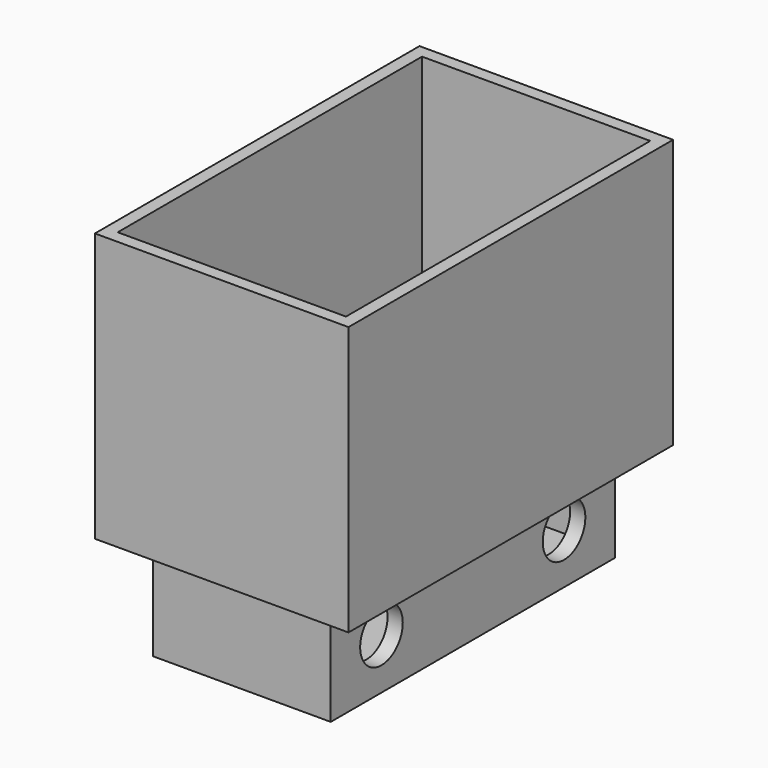
from build123d import *

# Parameters (mm, degrees)
F0_W         = 70
F0_H         = 20
F0_R         = 5.25
F1_DEPTH     = 17.5
F2_T         = -3
F3_W         = 80
F3_H         = 53
F4_DEPTH     = 25
F5_T         = 2.5
F5_T3_DEPTH  = 40
F5_T5_DEPTH  = 75
F5_T7_DEPTH  = 69
F5_T9_DEPTH  = 22
F5_T11_DEPTH = 34


# Not quite as in the source:
# - a shell that OpenCascade refuses in one call is made with other operations: the cavity is built on its own and cut out


with BuildPart() as f1:
    # F0 (on Right) → F1 (new body, symmetric)
    with BuildSketch(Plane.YZ):
        Rectangle(F0_W, F0_H)
        with Locations((-22.5, 0)):
            Circle(F0_R, mode=Mode.SUBTRACT)
        with Locations((22.5, 0)):
            Circle(F0_R, mode=Mode.SUBTRACT)
    extrude(amount=F1_DEPTH, both=True)

    # F2
    f2_openings = [f1.faces().sort_by_distance(p)[0] for p in [
        (0, 0, 10),
        (0, -27.75, 0),
        (0, 17.25, 0),
    ]]
    offset(amount=F2_T, openings=f2_openings)

    # F3 (on Right) → F4 (join, symmetric)
    with BuildSketch(Plane.YZ):
        with Locations((0, 36.5)):
            Rectangle(F3_W, F3_H)
    extrude(amount=F4_DEPTH, both=True)

    # F5: shell of thickness 2.5, made by hand


with BuildPart() as f5_core1:
    # F5_t2: copy of F1
    add(f1.part)

    # the walls: a layer under each face that stays
    f5_faces = [f5_core1.faces().sort_by_distance(p)[0] for p in [
        (-21.4285714286, -34.2857142857, 10),
        (-25, 0, 36.5),
        (0, -40, 36.5),
        (0, 40, 36.5),
        (25, 0, 36.5),
        (0, 35, 0),
        (17.5, 0, 0),
        (0, -35, 0),
        (-17.5, 0, 0),
        (0, 0, -10),
        (16, -27.75, 0),
        (16, 17.25, 0),
        (-16, -27.75, 0),
        (-16, 17.25, 0),
        (14.5, 0, 1.5),
        (-14.5, 0, 1.5),
        (0, 0, 10),
        (0, -32, 1.5),
        (0, 0, -7),
        (0, 32, 1.5),
    ]]
    thicken(f5_faces, amount=-F5_T, mode=Mode.SUBTRACT)

    # F5_s4 → F5_t3 (cut)
    with BuildSketch(Plane.YZ.offset(-20)):
        Polygon((35.025, 9.975), (35, 12.5), (32.5, 12.5), (32.5, 10), align=None)
        Polygon((-35.025, 9.975), (-35, 12.5), (-32.5, 12.5), (-32.5, 10), align=None)
    extrude(amount=F5_T3_DEPTH, mode=Mode.SUBTRACT)

    # F5_s6 → F5_t5 (cut)
    with BuildSketch(Plane.XZ.offset(-37.5)):
        Polygon((17.525, 9.975), (17.5, 12.5), (15, 12.5), (15, 10), align=None)
        Polygon((-17.525, 9.975), (-17.5, 12.5), (-15, 12.5), (-15, 10), align=None)
    extrude(amount=F5_T5_DEPTH, mode=Mode.SUBTRACT)

    # F5_s8 → F5_t7 (cut)
    with BuildSketch(Plane.XZ.offset(-34.5)):
        Polygon((14.475, 9.975), (17, 10), (17, 12.5), (14.5, 12.5), align=None)
        Polygon((14.475, -6.975), (17, -7), (17, -9.5), (14.5, -9.5), align=None)
        Polygon((-14.475, 9.975), (-17, 10), (-17, 12.5), (-14.5, 12.5), align=None)
        Polygon((-14.475, -6.975), (-17, -7), (-17, -9.5), (-14.5, -9.5), align=None)
    extrude(amount=F5_T7_DEPTH, mode=Mode.SUBTRACT)

    # F5_s10 → F5_t9 (cut)
    with BuildSketch(Plane.XY.offset(-9.5)):
        Polygon((14.475, -31.975), (17, -32), (17, -34.5), (14.5, -34.5), align=None)
        Polygon((14.475, 31.975), (17, 32), (17, 34.5), (14.5, 34.5), align=None)
        Polygon((-14.475, -31.975), (-17, -32), (-17, -34.5), (-14.5, -34.5), align=None)
        Polygon((-14.475, 31.975), (-17, 32), (-17, 34.5), (-14.5, 34.5), align=None)
    extrude(amount=F5_T9_DEPTH, mode=Mode.SUBTRACT)

    # F5_s12 → F5_t11 (cut)
    with BuildSketch(Plane.YZ.offset(-17)):
        Polygon((-31.975, 9.975), (-32, 12.5), (-34.5, 12.5), (-34.5, 10), align=None)
        Polygon((31.975, 9.975), (32, 12.5), (34.5, 12.5), (34.5, 10), align=None)
        Polygon((-31.975, -6.975), (-34.5, -7), (-34.5, -9.5), (-32, -9.5), align=None)
        Polygon((31.975, -6.975), (32, -9.5), (34.5, -9.5), (34.5, -7), align=None)
    extrude(amount=F5_T11_DEPTH, mode=Mode.SUBTRACT)


with BuildPart() as f1_1:
    add(f1.part)

    # what is left inside the walls is the cavity
    f5_cavity = [f5_core1.part.solids().sort_by_distance(p)[0] for p in [
        (22.475, 0, 29.333333),
    ]]
    add(f5_cavity, mode=Mode.SUBTRACT)


solid = f1_1.part
